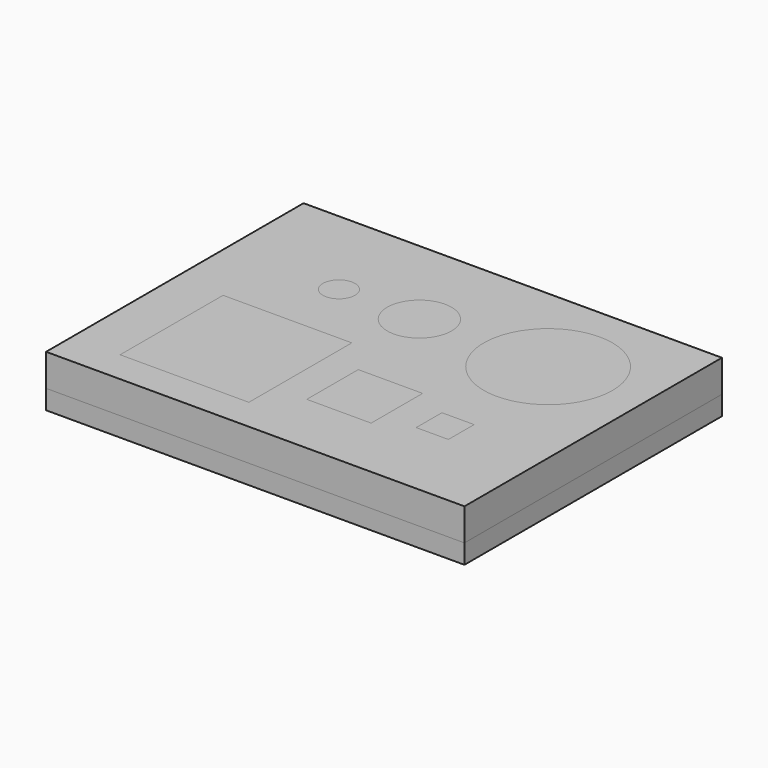
from build123d import *

# Parameters (mm, degrees)
F0_W     = 65
F0_H     = 50
F0_W_2   = 20
F0_H_2   = 20
F0_W_3   = 10
F0_H_3   = 10
F0_W_4   = 5
F0_H_4   = 5
F0_R     = 2.5
F0_R_2   = 5
F0_R_3   = 10
F1_DEPTH = 5
F2_DEPTH = 5
F3_DEPTH = 3


with BuildPart() as f1:
    # F0 (on Top) → F1 (new body)
    with BuildSketch(Plane.XY):
        Rectangle(F0_W, F0_H)
        with Locations((-15, -10)):
            Rectangle(F0_W_2, F0_H_2, mode=Mode.SUBTRACT)
        with Locations((5, -10)):
            Rectangle(F0_W_3, F0_H_3, mode=Mode.SUBTRACT)
        with Locations((17.5, -10)):
            Rectangle(F0_W_4, F0_H_4, mode=Mode.SUBTRACT)
        with Locations((-15, 10)):
            Circle(F0_R, mode=Mode.SUBTRACT)
        with Locations((-2.5, 10)):
            Circle(F0_R_2, mode=Mode.SUBTRACT)
        with Locations((17.5, 10)):
            Circle(F0_R_3, mode=Mode.SUBTRACT)
    extrude(amount=F1_DEPTH)


with BuildPart() as f2:
    # F0 (on Top) → F2 (new body)
    with BuildSketch(Plane.XY):
        with Locations((-15, -10)):
            Rectangle(F0_W_2, F0_H_2)
    extrude(amount=F2_DEPTH)



with BuildPart() as f2b:
    # F0 (on Top) → F2, piece 2 (new body)
    with BuildSketch(Plane.XY):
        with Locations((5, -10)):
            Rectangle(F0_W_3, F0_H_3)
    extrude(amount=F2_DEPTH)


with BuildPart() as f2c:
    # F0 (on Top) → F2, piece 3 (new body)
    with BuildSketch(Plane.XY):
        with Locations((17.5, -10)):
            Rectangle(F0_W_4, F0_H_4)
    extrude(amount=F2_DEPTH)


with BuildPart() as f2d:
    # F0 (on Top) → F2, piece 4 (new body)
    with BuildSketch(Plane.XY):
        with Locations((17.5, 10)):
            Circle(F0_R_3)
    extrude(amount=F2_DEPTH)


with BuildPart() as f2e:
    # F0 (on Top) → F2, piece 5 (new body)
    with BuildSketch(Plane.XY):
        with Locations((-2.5, 10)):
            Circle(F0_R_2)
    extrude(amount=F2_DEPTH)


with BuildPart() as f2f:
    # F0 (on Top) → F2, piece 6 (new body)
    with BuildSketch(Plane.XY):
        with Locations((-15, 10)):
            Circle(F0_R)
    extrude(amount=F2_DEPTH)


with BuildPart() as f2_1:
    add(f2.part)

    add(f2b.part)  # F3 merges F2b

    add(f2c.part)  # F3 merges F2c

    add(f2d.part)  # F3 merges F2d

    add(f2e.part)  # F3 merges F2e

    add(f2f.part)  # F3 merges F2f
    # F0 (on Top) → F3 (join)
    with BuildSketch(Plane.XY):
        Rectangle(F0_W, F0_H)
        with Locations((-15, -10)):
            Rectangle(F0_W_2, F0_H_2, mode=Mode.SUBTRACT)
        with Locations((5, -10)):
            Rectangle(F0_W_3, F0_H_3, mode=Mode.SUBTRACT)
        with Locations((17.5, -10)):
            Rectangle(F0_W_4, F0_H_4, mode=Mode.SUBTRACT)
        with Locations((-15, 10)):
            Circle(F0_R, mode=Mode.SUBTRACT)
        with Locations((-2.5, 10)):
            Circle(F0_R_2, mode=Mode.SUBTRACT)
        with Locations((17.5, 10)):
            Circle(F0_R_3, mode=Mode.SUBTRACT)
        with Locations((-15, -10)):
            Rectangle(F0_W_2, F0_H_2)
        with Locations((-15, 10)):
            Circle(F0_R)
        with Locations((-2.5, 10)):
            Circle(F0_R_2)
        with Locations((5, -10)):
            Rectangle(F0_W_3, F0_H_3)
        with Locations((17.5, -10)):
            Rectangle(F0_W_4, F0_H_4)
        with Locations((17.5, 10)):
            Circle(F0_R_3)
    extrude(amount=-F3_DEPTH)


solid = Compound([f1.part, f2_1.part])
